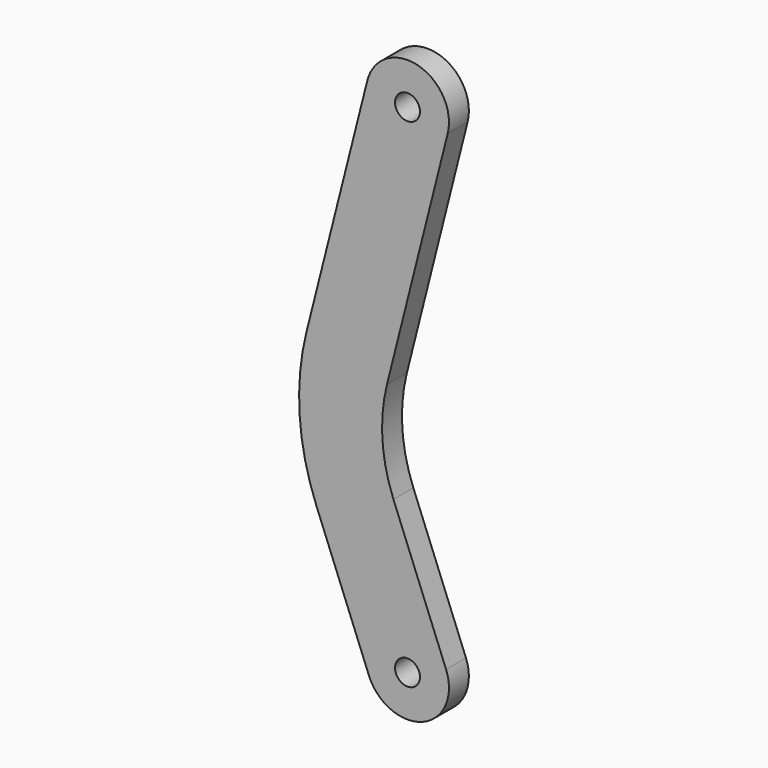
from build123d import *

# Parameters (mm, degrees)
F1_DEPTH = 3
F2_D     = 3


# Not quite as in the source:
# - a feature of the source that left no trace in its solid (it failed there, or was rolled back) is left out


with BuildPart() as f1:
    # F0 (on Front) → F1 (new body)
    with BuildSketch(Plane.XZ):
        with BuildLine():
            ThreePointArc((6.3713843202, -7.1733870463), (5.0414339245, -1.2687792727), (5.5912292227, 4.7587315024))
            Line((5.5912292227, 4.7587315024), (12.9146554895, 33.77647678))
            ThreePointArc((12.9146554895, 33.77647678), (9.290190371, 39.8479883385), (3.2186788125, 36.22352322))
            Line((3.2186788125, 36.22352322), (-4.1047474542, 7.2057779424))
            ThreePointArc((-4.1047474542, 7.2057779424), (-4.9372598224, -1.9212140236), (-2.9234191128, -10.8621035089))
            Line((-2.9234191128, -10.8621035089), (3.4192654345, -26.8443582313))
            ThreePointArc((3.4192654345, -26.8443582313), (9.9110253823, -29.6474017165), (12.7140688675, -23.1556417687))
            Line((12.7140688675, -23.1556417687), (6.3713843202, -7.1733870463))
        make_face()
    extrude(amount=F1_DEPTH)

    # F2 (through all)
    with Locations(Plane(origin=(0, 0, 0), x_dir=(1, 0, 0), z_dir=(0, 1, 0))):
        with Locations((8.066667151, -35), (8.066667151, 25)):
            Hole(F2_D / 2)


solid = f1.part
